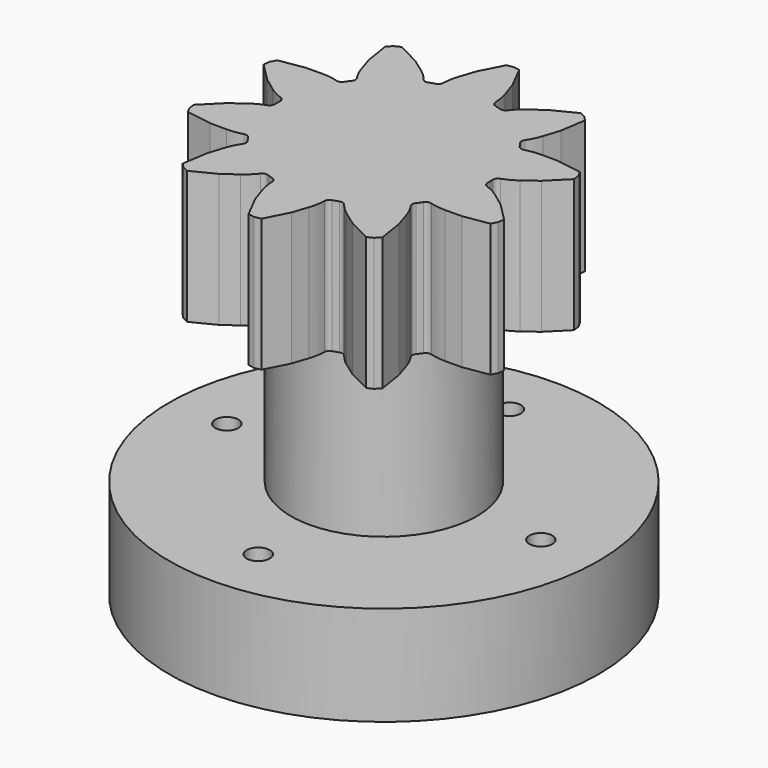
from build123d import *

# Parameters (mm, degrees)
F1_DEPTH  = 6.35
F2_R      = 0.254
F3_R      = 2.54
F4_R      = 4.445
F5_DEPTH  = 12.7
F6_R      = 10.25
F7_DEPTH  = 4.7625
F8_R      = 5
F9_DEPTH  = 1
F10_R     = 0.55
F11_DEPTH = 4.7625


# Not quite as in the source:
# - a feature names something its author has since deleted; it is built from what else it names


with BuildPart() as f1:
    # F0 (on Top) → F1 (new body)
    with BuildSketch(Plane.XY):
        with BuildLine():
            ThreePointArc((5.0687244587, -0.3382785271), (5.0771803321, -0.1692331969), (5.08, 0))
            ThreePointArc((5.08, 0), (5.0771803321, 0.1692331969), (5.0687244587, 0.3382785271))
            ThreePointArc((5.0687244587, 0.3382785271), (4.9881979125, 0.9613956446), (4.8313671028, 1.5698063314))
            ThreePointArc((4.8313671028, 1.5698063314), (4.6006310641, 2.1542037537), (4.2995193563, 2.7056484075))
            ThreePointArc((4.2995193563, 2.7056484075), (4.1098063314, 2.9859490816), (3.9018490975, 3.252994562))
            ThreePointArc((3.9018490975, 3.252994562), (3.470442701, 3.7097745833), (2.9859490816, 4.1098063314))
            ThreePointArc((2.9859490816, 4.1098063314), (2.4557795188, 4.4469705368), (1.8880439951, 4.716109612))
            ThreePointArc((1.8880439951, 4.716109612), (1.5698063314, 4.8313671028), (1.2446, 4.9251772395))
            ThreePointArc((1.2446, 4.9251772395), (0.6270963337, 5.0411457218), (0, 5.08))
            ThreePointArc((0, 5.08), (-0.6270963337, 5.0411457218), (-1.2446, 4.9251772395))
            ThreePointArc((-1.2446, 4.9251772395), (-1.5698063314, 4.8313671028), (-1.8880439951, 4.716109612))
            ThreePointArc((-1.8880439951, 4.716109612), (-2.4557795188, 4.4469705368), (-2.9859490816, 4.1098063314))
            ThreePointArc((-2.9859490816, 4.1098063314), (-3.470442701, 3.7097745833), (-3.9018490975, 3.252994562))
            ThreePointArc((-3.9018490975, 3.252994562), (-4.1098063314, 2.9859490816), (-4.2995193563, 2.7056484075))
            ThreePointArc((-4.2995193563, 2.7056484075), (-4.6006310641, 2.1542037537), (-4.8313671028, 1.5698063314))
            ThreePointArc((-4.8313671028, 1.5698063314), (-4.9881979125, 0.9613956446), (-5.0687244587, 0.3382785271))
            ThreePointArc((-5.0687244587, 0.3382785271), (-5.08, 0), (-5.0687244587, -0.3382785271))
            ThreePointArc((-5.0687244587, -0.3382785271), (-4.9881979125, -0.9613956446), (-4.8313671028, -1.5698063314))
            ThreePointArc((-4.8313671028, -1.5698063314), (-4.6006310641, -2.1542037537), (-4.2995193563, -2.7056484075))
            ThreePointArc((-4.2995193563, -2.7056484075), (-4.1098063314, -2.9859490816), (-3.9018490975, -3.252994562))
            ThreePointArc((-3.9018490975, -3.252994562), (-3.470442701, -3.7097745833), (-2.9859490816, -4.1098063314))
            ThreePointArc((-2.9859490816, -4.1098063314), (-2.4557795188, -4.4469705368), (-1.8880439951, -4.716109612))
            ThreePointArc((-1.8880439951, -4.716109612), (-1.5698063314, -4.8313671028), (-1.2446, -4.9251772395))
            ThreePointArc((-1.2446, -4.9251772395), (-0.6270963337, -5.0411457218), (0, -5.08))
            ThreePointArc((0, -5.08), (0.6270963337, -5.0411457218), (1.2446, -4.9251772395))
            ThreePointArc((1.2446, -4.9251772395), (1.5698063314, -4.8313671028), (1.8880439951, -4.716109612))
            ThreePointArc((1.8880439951, -4.716109612), (2.4557795188, -4.4469705368), (2.9859490816, -4.1098063314))
            ThreePointArc((2.9859490816, -4.1098063314), (3.470442701, -3.7097745833), (3.9018490975, -3.252994562))
            ThreePointArc((3.9018490975, -3.252994562), (4.1098063314, -2.9859490816), (4.2995193563, -2.7056484075))
            ThreePointArc((4.2995193563, -2.7056484075), (4.6006310641, -2.1542037537), (4.8313671028, -1.5698063314))
            ThreePointArc((4.8313671028, -1.5698063314), (4.9881979125, -0.9613956446), (5.0687244587, -0.3382785271))
        make_face()
        with BuildLine():
            ThreePointArc((4.8313671028, 1.5698063314), (4.9881979125, 0.9613956446), (5.0687244587, 0.3382785271))
            Line((5.0687244587, 0.3382785271), (5.215969654, 0.3861213912))
            Line((5.215969654, 0.3861213912), (4.8313671028, 1.5698063314))
        make_face()
        with BuildLine():
            Line((5.215969654, -0.3861213912), (5.0687244587, -0.3382785271))
            ThreePointArc((5.0687244587, -0.3382785271), (4.9881979125, -0.9613956446), (4.8313671028, -1.5698063314))
            Line((4.8313671028, -1.5698063314), (5.215969654, -0.3861213912))
        make_face()
        with BuildLine():
            ThreePointArc((4.2995193563, 2.7056484075), (4.6006310641, 2.1542037537), (4.8313671028, 1.5698063314))
            Line((4.8313671028, 1.5698063314), (4.4467645516, 2.7534912716))
            Line((4.4467645516, 2.7534912716), (4.2995193563, 2.7056484075))
        make_face()
        Polygon((4.4467645516, 2.7534912716), (4.8313671028, 1.5698063314), (5.215969654, 0.3861213912), (5.5783221867, 0.5038568661), (6.54764431, 1.2194158234), (7.4137095406, 2.0883745659), (7.3722313758, 2.3953831792), (7.2253327808, 2.6681386183), (6.0139101573, 2.8620806383), (4.8091170843, 2.8712267465), align=None)
        with BuildLine():
            Line((4.4467645516, -2.7534912716), (4.8313671028, -1.5698063314))
            ThreePointArc((4.8313671028, -1.5698063314), (4.6006310641, -2.1542037537), (4.2995193563, -2.7056484075))
            Line((4.2995193563, -2.7056484075), (4.4467645516, -2.7534912716))
        make_face()
        Polygon((5.215969654, -0.3861213912), (4.8313671028, -1.5698063314), (4.4467645516, -2.7534912716), (4.8091170843, -2.8712267465), (6.0139101573, -2.8620806383), (7.2253327808, -2.6681386183), (7.3722313758, -2.3953831792), (7.4137095406, -2.0883745659), (6.54764431, -1.2194158234), (5.5783221867, -0.5038568661), align=None)
        with BuildLine():
            ThreePointArc((2.9859490816, 4.1098063314), (3.470442701, 3.7097745833), (3.9018490975, 3.252994562))
            Line((3.9018490975, 3.252994562), (3.9928516328, 3.3782488064))
            Line((3.9928516328, 3.3782488064), (2.9859490816, 4.1098063314))
        make_face()
        with BuildLine():
            Line((3.9928516328, -3.3782488064), (3.9018490975, -3.252994562))
            ThreePointArc((3.9018490975, -3.252994562), (3.470442701, -3.7097745833), (2.9859490816, -4.1098063314))
            Line((2.9859490816, -4.1098063314), (3.9928516328, -3.3782488064))
        make_face()
        with BuildLine():
            ThreePointArc((1.8880439951, 4.716109612), (2.4557795188, 4.4469705368), (2.9859490816, 4.1098063314))
            Line((2.9859490816, 4.1098063314), (1.9790465304, 4.8413638564))
            Line((1.9790465304, 4.8413638564), (1.8880439951, 4.716109612))
        make_face()
        Polygon((1.9790465304, 4.8413638564), (2.9859490816, 4.1098063314), (3.9928516328, 3.3782488064), (4.216797814, 3.6864842813), (4.5804008825, 4.835136887), (4.7703012386, 6.0471996472), (4.5562895632, 6.2711945792), (4.2771244788, 6.405513537), (3.1830667298, 5.8503595747), (2.2029927116, 5.1495993313), align=None)
        with BuildLine():
            Line((1.9790465304, -4.8413638564), (2.9859490816, -4.1098063314))
            ThreePointArc((2.9859490816, -4.1098063314), (2.4557795188, -4.4469705368), (1.8880439951, -4.716109612))
            Line((1.8880439951, -4.716109612), (1.9790465304, -4.8413638564))
        make_face()
        Polygon((3.9928516328, -3.3782488064), (2.9859490816, -4.1098063314), (1.9790465304, -4.8413638564), (2.2029927116, -5.1495993313), (3.1830667298, -5.8503595747), (4.2771244788, -6.405513537), (4.5562895632, -6.2711945792), (4.7703012386, -6.0471996472), (4.5804008825, -4.835136887), (4.216797814, -3.6864842813), align=None)
        with BuildLine():
            ThreePointArc((0, 5.08), (0.6270963337, 5.0411457218), (1.2446, 4.9251772395))
            Line((1.2446, 4.9251772395), (1.2446, 5.08))
            Line((1.2446, 5.08), (0, 5.08))
        make_face()
        with BuildLine():
            Line((1.2446, -5.08), (1.2446, -4.9251772395))
            ThreePointArc((1.2446, -4.9251772395), (0.6270963337, -5.0411457218), (0, -5.08))
            Line((0, -5.08), (1.2446, -5.08))
        make_face()
        with BuildLine():
            ThreePointArc((-1.2446, 4.9251772395), (-0.6270963337, 5.0411457218), (0, 5.08))
            Line((0, 5.08), (-1.2446, 5.08))
            Line((-1.2446, 5.08), (-1.2446, 4.9251772395))
        make_face()
        Polygon((-1.2446, 5.08), (0, 5.08), (1.2446, 5.08), (1.2446, 5.461), (0.8636, 6.604), (0.3048, 7.6962), (0, 7.7516228), (-0.3048, 7.6962), (-0.8636, 6.604), (-1.2446, 5.461), align=None)
        with BuildLine():
            Line((-1.2446, -5.08), (0, -5.08))
            ThreePointArc((0, -5.08), (-0.6270963337, -5.0411457218), (-1.2446, -4.9251772395))
            Line((-1.2446, -4.9251772395), (-1.2446, -5.08))
        make_face()
        Polygon((1.2446, -5.08), (0, -5.08), (-1.2446, -5.08), (-1.2446, -5.461), (-0.8636, -6.604), (-0.3048, -7.6962), (0, -7.7516228), (0.3048, -7.6962), (0.8636, -6.604), (1.2446, -5.461), align=None)
        with BuildLine():
            ThreePointArc((-2.9859490816, 4.1098063314), (-2.4557795188, 4.4469705368), (-1.8880439951, 4.716109612))
            Line((-1.8880439951, 4.716109612), (-1.9790465304, 4.8413638564))
            Line((-1.9790465304, 4.8413638564), (-2.9859490816, 4.1098063314))
        make_face()
        with BuildLine():
            Line((-1.9790465304, -4.8413638564), (-1.8880439951, -4.716109612))
            ThreePointArc((-1.8880439951, -4.716109612), (-2.4557795188, -4.4469705368), (-2.9859490816, -4.1098063314))
            Line((-2.9859490816, -4.1098063314), (-1.9790465304, -4.8413638564))
        make_face()
        Polygon((-3.9928516328, 3.3782488064), (-2.9859490816, 4.1098063314), (-1.9790465304, 4.8413638564), (-2.2029927116, 5.1495993313), (-3.1830667298, 5.8503595747), (-4.2771244788, 6.405513537), (-4.5562895632, 6.2711945792), (-4.7703012386, 6.0471996472), (-4.5804008825, 4.835136887), (-4.216797814, 3.6864842813), align=None)
        with BuildLine():
            ThreePointArc((-3.9018490975, 3.252994562), (-3.470442701, 3.7097745833), (-2.9859490816, 4.1098063314))
            Line((-2.9859490816, 4.1098063314), (-3.9928516328, 3.3782488064))
            Line((-3.9928516328, 3.3782488064), (-3.9018490975, 3.252994562))
        make_face()
        with BuildLine():
            Line((-3.9928516328, -3.3782488064), (-2.9859490816, -4.1098063314))
            ThreePointArc((-2.9859490816, -4.1098063314), (-3.470442701, -3.7097745833), (-3.9018490975, -3.252994562))
            Line((-3.9018490975, -3.252994562), (-3.9928516328, -3.3782488064))
        make_face()
        Polygon((-1.9790465304, -4.8413638564), (-2.9859490816, -4.1098063314), (-3.9928516328, -3.3782488064), (-4.216797814, -3.6864842813), (-4.5804008825, -4.835136887), (-4.7703012386, -6.0471996472), (-4.5562895632, -6.2711945792), (-4.2771244788, -6.405513537), (-3.1830667298, -5.8503595747), (-2.2029927116, -5.1495993313), align=None)
        with BuildLine():
            ThreePointArc((-4.8313671028, 1.5698063314), (-4.6006310641, 2.1542037537), (-4.2995193563, 2.7056484075))
            Line((-4.2995193563, 2.7056484075), (-4.4467645516, 2.7534912716))
            Line((-4.4467645516, 2.7534912716), (-4.8313671028, 1.5698063314))
        make_face()
        with BuildLine():
            Line((-4.4467645516, -2.7534912716), (-4.2995193563, -2.7056484075))
            ThreePointArc((-4.2995193563, -2.7056484075), (-4.6006310641, -2.1542037537), (-4.8313671028, -1.5698063314))
            Line((-4.8313671028, -1.5698063314), (-4.4467645516, -2.7534912716))
        make_face()
        Polygon((-5.215969654, 0.3861213912), (-4.8313671028, 1.5698063314), (-4.4467645516, 2.7534912716), (-4.8091170843, 2.8712267465), (-6.0139101573, 2.8620806383), (-7.2253327808, 2.6681386183), (-7.3722313758, 2.3953831792), (-7.4137095406, 2.0883745659), (-6.54764431, 1.2194158234), (-5.5783221867, 0.5038568661), align=None)
        with BuildLine():
            ThreePointArc((-5.0687244587, 0.3382785271), (-4.9881979125, 0.9613956446), (-4.8313671028, 1.5698063314))
            Line((-4.8313671028, 1.5698063314), (-5.215969654, 0.3861213912))
            Line((-5.215969654, 0.3861213912), (-5.0687244587, 0.3382785271))
        make_face()
        with BuildLine():
            Line((-5.215969654, -0.3861213912), (-4.8313671028, -1.5698063314))
            ThreePointArc((-4.8313671028, -1.5698063314), (-4.9881979125, -0.9613956446), (-5.0687244587, -0.3382785271))
            Line((-5.0687244587, -0.3382785271), (-5.215969654, -0.3861213912))
        make_face()
        Polygon((-4.4467645516, -2.7534912716), (-4.8313671028, -1.5698063314), (-5.215969654, -0.3861213912), (-5.5783221867, -0.5038568661), (-6.54764431, -1.2194158234), (-7.4137095406, -2.0883745659), (-7.3722313758, -2.3953831792), (-7.2253327808, -2.6681386183), (-6.0139101573, -2.8620806383), (-4.8091170843, -2.8712267465), align=None)
    extrude(amount=F1_DEPTH)

    # F2
    f2_edges = [f1.edges().sort_by_distance(p)[0] for p in [
        (5.068724, -0.338279, 3.175),
        (4.299519, -2.705648, 3.175),
        (3.901849, -3.252995, 3.175),
        (1.888044, -4.71611, 3.175),
        (1.2446, -4.925177, 3.175),
        (-1.2446, -4.925177, 3.175),
        (-1.888044, -4.71611, 3.175),
        (-3.901849, -3.252995, 3.175),
        (-4.299519, -2.705648, 3.175),
        (-5.068724, -0.338279, 3.175),
        (-5.068724, 0.338279, 3.175),
        (-4.299519, 2.705648, 3.175),
        (-3.901849, 3.252995, 3.175),
        (-1.888044, 4.71611, 3.175),
        (-1.2446, 4.925177, 3.175),
        (1.2446, 4.925177, 3.175),
        (1.888044, 4.71611, 3.175),
        (3.901849, 3.252995, 3.175),
        (4.299519, 2.705648, 3.175),
        (5.068724, 0.338279, 3.175),
    ]]
    fillet(f2_edges, radius=F2_R)

    # F3
    f3_edges = [f1.edges().sort_by_distance(p)[0] for p in [
        (1.2446, 5.461, 3.175),
        (-1.2446, 5.461, 3.175),
        (-2.202993, 5.149599, 3.175),
        (-4.809117, 2.871227, 3.175),
        (-4.216798, 3.686484, 3.175),
        (-5.578322, 0.503857, 3.175),
        (-5.578322, -0.503857, 3.175),
        (-4.809117, -2.871227, 3.175),
        (-4.216798, -3.686484, 3.175),
        (-2.202993, -5.149599, 3.175),
        (-1.2446, -5.461, 3.175),
        (1.2446, -5.461, 3.175),
        (2.202993, -5.149599, 3.175),
        (4.809117, -2.871227, 3.175),
        (4.216798, -3.686484, 3.175),
        (5.578322, -0.503857, 3.175),
        (4.216798, 3.686484, 3.175),
        (2.202993, 5.149599, 3.175),
        (4.809117, 2.871227, 3.175),
        (5.578322, 0.503857, 3.175),
    ]]
    fillet(f3_edges, radius=F3_R)

    # F4 (on face) → F5 (join)
    with BuildSketch(Plane(origin=(0, 0, 0), x_dir=(1, 0, 0), z_dir=(0, 0, -1))):
        Circle(F4_R)
    extrude(amount=F5_DEPTH)

    # F6 (on face) → F7 (join)
    with BuildSketch(Plane(origin=(0, 0, -12.7), x_dir=(1, 0, 0), z_dir=(0, 0, -1))):
        Circle(F6_R)
    extrude(amount=-F7_DEPTH)

    # F8 (on face) → F9 (cut)
    with BuildSketch(Plane(origin=(0, 0, -12.7), x_dir=(1, 0, 0), z_dir=(0, 0, -1))):
        Circle(F8_R)
    extrude(amount=-F9_DEPTH, mode=Mode.SUBTRACT)

    # F10 (on face) → F11 (cut, through all)
    with BuildSketch(Plane(origin=(0, 0, -12.7), x_dir=(1, 0, 0), z_dir=(0, 0, -1))):
        with Locations((7.5, 0)):
            Circle(F10_R)
        with Locations((0, 7.5)):
            Circle(F10_R)
        with Locations((-7.5, 0)):
            Circle(F10_R)
        with Locations((0, -7.5)):
            Circle(F10_R)
    extrude(amount=-F11_DEPTH, mode=Mode.SUBTRACT)


solid = f1.part
